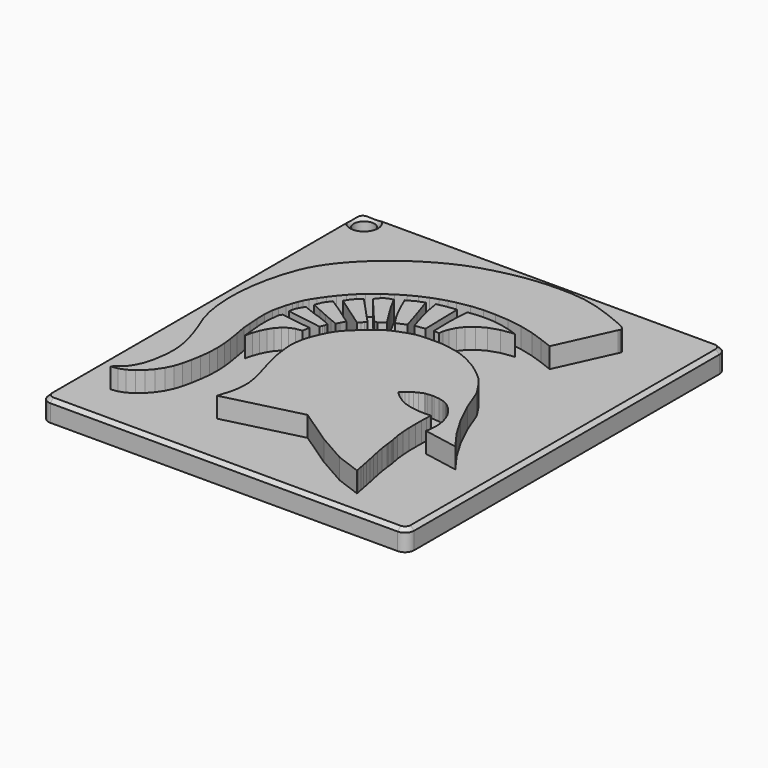
from build123d import *

# Parameters (mm, degrees)
F1_DEPTH     = 22.86
F2_W         = 203.2
F2_H         = 222.25
F2_R         = 5.715
F3_DEPTH     = 11.61275
F4_R         = 5.08
F5_T1_DEPTH  = 212.09
F5_T3_DEPTH  = 193.04
F5_T10_ANGLE = 90
F5_T12_ANGLE = 90
F5_T14_ANGLE = 90
F5_T16_ANGLE = 90


# Not quite as in the source:
# - a fillet or chamfer that OpenCascade refuses, or shapes differently, is made with other operations: its cross-section is extruded or revolved along the edge and cut away or added


with BuildPart() as f1:
    # F0 (on Top) → F1 (new body)
    with BuildSketch(Plane.XY):
        Polygon((-28.5374334, -76.846176), (-28.6309054, -77.130148), (13.3961886, -66.648838), (32.9714606, -79.89316), (49.1756446, -89.098628), (62.7590566, -94.076012), (62.6846346, -93.659706), (62.4725446, -92.483178), (62.1321846, -90.644726), (61.6787946, -88.24849), (61.1235506, -85.393022), (60.4773746, -82.180684), (59.7552526, -78.713584), (58.9681066, -75.093576), (58.1662286, -70.861428), (57.6066666, -66.742818), (57.5294506, -66.16954), (57.4758566, -65.83426), (57.4166746, -65.359026), (57.3242186, -64.361568), (57.1421006, -62.889638), (57.0415166, -62.196472), (56.8860686, -61.420756), (56.1268626, -57.560718), (55.6541686, -53.167534), (55.4100746, -48.56226), (55.3384466, -44.069762), (55.3811186, -40.012874), (55.4817026, -36.713922), (55.5850806, -34.497772), (55.6318166, -33.687512), (55.2985686, -33.722056), (54.3544506, -33.79216), (52.8840446, -33.846262), (50.9742186, -33.833816), (48.7044746, -33.701482), (46.1634586, -33.398206), (43.4334666, -32.874712), (40.5990806, -32.078168), (38.7895846, -31.333948), (37.0298726, -30.374844), (35.3803966, -29.295598), (33.8975446, -28.197556), (32.6407526, -27.172412), (31.6704726, -26.32075), (31.0451246, -25.73909), (30.8246526, -25.524206), (30.9389526, -25.358598), (31.3011566, -24.901144), (31.9435226, -24.207978), (32.8929746, -23.332948), (34.1802466, -22.331172), (35.8350566, -21.259038), (37.8868686, -20.171918), (40.3661626, -19.125946), (40.5137366, -19.106388), (40.9186126, -19.057112), (41.5165286, -18.988278), (42.2472866, -18.911062), (43.0491646, -18.833846), (43.8579006, -18.767298), (44.6145666, -18.72361), (45.2566786, -18.713704), (48.4814626, -19.051524), (51.0321306, -19.726656), (52.7105626, -20.386548), (53.3140666, -20.68576), (53.5868626, -20.857972), (54.3313366, -21.377656), (55.4281086, -22.244304), (56.7661806, -23.461218), (58.2269346, -25.02916), (59.6945466, -26.950416), (61.0544626, -29.225494), (62.1928906, -31.857696), (62.9932446, -34.675572), (63.4341886, -37.343588), (63.5942086, -39.789354), (63.5489966, -41.944798), (63.3765306, -43.740578), (63.1573286, -45.108622), (62.9686066, -45.981112), (62.8885966, -46.286928), (82.0409586, -49.814734), (74.8403126, -39.931594), (68.4324006, -29.101288), (62.7798846, -17.36344), (57.8492366, -4.759706), (57.6465446, -4.430522), (57.0872366, -3.536188), (56.2449726, -2.214626), (55.1908726, -0.606298), (53.9960566, 1.15316), (52.7367246, 2.924302), (51.4801866, 4.566666), (50.3031506, 5.943346), (49.0821726, 7.149084), (47.6171006, 8.444484), (46.0323946, 9.7536), (44.4535306, 10.997946), (43.0062386, 12.10183), (41.8172646, 12.986512), (41.0110686, 13.573506), (40.7146506, 13.78585), (40.4004526, 13.974572), (39.5378686, 14.48435), (38.2356106, 15.23111), (36.6107726, 16.131032), (34.7738446, 17.101312), (32.8393806, 18.057622), (30.9193946, 18.916396), (29.1294566, 19.594322), (27.6880066, 20.013168), (25.9600446, 20.42795), (24.0928906, 20.824952), (22.2338646, 21.185632), (20.5305406, 21.495766), (19.1302386, 21.73859), (18.1838346, 21.895562), (17.8353466, 21.95068), (17.4492666, 21.959062), (16.3702746, 21.9837), (14.7385786, 22.008338), (12.6992126, 22.018244), (10.3895906, 21.996146), (7.9519526, 21.925788), (5.5280306, 21.79066), (3.2610806, 21.574506), (1.4335506, 21.14296), (-0.5725414, 20.535646), (-2.6286714, 19.821652), (-4.6019974, 19.076162), (-6.3645034, 18.36928), (-7.7851254, 17.775174), (-8.7335614, 17.36598), (-9.0779854, 17.213072), (-9.6428814, 16.816324), (-11.1656114, 15.710916), (-13.3926834, 14.035278), (-16.0716214, 11.924284), (-18.9474094, 9.511284), (-21.7668094, 6.93293), (-24.2775994, 4.322826), (-26.2234934, 1.8161), (-27.9542494, -1.10109), (-29.5971214, -4.418076), (-31.0604154, -7.947406), (-32.2524374, -11.504168), (-32.7774554, -13.953998), (-33.1589634, -16.706088), (-33.3906114, -18.95094), (-33.4690974, -19.879818), (-33.4416654, -20.324826), (-33.3535274, -21.549868), (-33.1937614, -23.392384), (-32.9537314, -25.686766), (-32.6260714, -28.26639), (-32.2001134, -30.968696), (-31.6667134, -33.628584), (-31.0177434, -36.081462), (-30.7104034, -37.391594), (-30.2529494, -39.114222), (-29.6890694, -41.127426), (-29.0637214, -43.307762), (-28.4203394, -45.529246), (-27.8013414, -47.670466), (-27.2514314, -49.609248), (-26.8160754, -51.22037), (-26.1864094, -54.030372), (-25.7480054, -56.559196), (-25.4904494, -58.384694), (-25.4063754, -59.087512), (-25.4035814, -59.9821), (-25.4391414, -62.184026), (-25.5829054, -64.966596), (-25.8996434, -67.601084), (-26.1820914, -68.897754), (-26.5681714, -70.392798), (-27.0157194, -71.973694), (-27.4805394, -73.523856), (-27.9184354, -74.929746), (-28.2852114, -76.074778), align=None)
    extrude(amount=F1_DEPTH)


with BuildPart() as f1b:
    # F0 (on Top) → F1, piece 2 (new body)
    with BuildSketch(Plane.XY):
        Polygon((-55.0672254, -19.514566), (-54.5256974, -25.240234), (-53.4987754, -21.424646), (-52.2559534, -17.902174), (-50.7537974, -14.729968), (-48.9501434, -11.96975), (-46.8018114, -9.678162), (-44.2648594, -7.915656), (-41.2950914, -6.740144), (-37.8485654, -6.211062), (-37.1348254, -2.21869), (-53.8833314, 0.132334), (-54.8109394, -0.865378), (-55.6473614, -7.671562), (-55.5866554, -13.773404), align=None)
    extrude(amount=F1_DEPTH)


with BuildPart() as f1c:
    # F0 (on Top) → F1, piece 3 (new body)
    with BuildSketch(Plane.XY):
        Polygon((-53.6326334, 5.551932), (-53.8132274, 4.480052), (-34.4269314, 1.34493), (-33.8414614, 2.590546), (-33.4746854, 3.615944), (-33.2473554, 4.503166), (-33.0723494, 5.335778), (-35.2277934, 6.342888), (-37.6199654, 7.368032), (-40.4640034, 8.429244), (-43.9765694, 9.54024), (-50.6765814, 12.177522), (-52.3867634, 9.326372), (-53.0662134, 7.85876), (-53.4327354, 6.639306), align=None)
    extrude(amount=F1_DEPTH)


with BuildPart() as f1d:
    # F0 (on Top) → F1, piece 4 (new body)
    with BuildSketch(Plane.XY):
        Polygon((-40.1444714, 20.660868), (-44.7609214, 23.652734), (-47.4703394, 20.017232), (-49.0382814, 15.954756), (-44.0540394, 13.701776), (-39.1424414, 11.495532), (-34.5991434, 9.523476), (-30.7213254, 7.97306), (-30.4965354, 8.382254), (-30.2940974, 8.743696), (-30.0916594, 9.10209), (-29.8696634, 9.504172), (-29.6080434, 9.9949), (-29.2841934, 10.621772), (-28.8788094, 11.429238), (-28.3690314, 12.463018), (-32.2013834, 15.161006), (-36.0418634, 17.862296), align=None)
    extrude(amount=F1_DEPTH)


with BuildPart() as f1e:
    # F0 (on Top) → F1, piece 5 (new body)
    with BuildSketch(Plane.XY):
        Polygon((-40.5564594, 28.533852), (-41.6959034, 26.717244), (-24.0929414, 14.529816), (-22.8099874, 15.813024), (-21.7061034, 16.84655), (-21.0284314, 18.022062), (-35.5678994, 33.631124), (-37.6489214, 32.02559), (-39.2582654, 30.313884), align=None)
    extrude(amount=F1_DEPTH)


with BuildPart() as f1f:
    # F0 (on Top) → F1, piece 6 (new body)
    with BuildSketch(Plane.XY):
        Polygon((-22.1058994, 35.819334), (-25.0190254, 41.327324), (-27.6359874, 40.711374), (-29.6342054, 39.529004), (-31.2135774, 37.963602), (-32.5734934, 36.196778), (-19.2466214, 20.302728), (-18.5366914, 20.20316), (-18.0157374, 20.166076), (-17.5956214, 20.162012), (-17.1793154, 20.160488), (-13.9009374, 22.511512), (-16.6253414, 26.879804), (-19.3332354, 31.160212), align=None)
    extrude(amount=F1_DEPTH)


with BuildPart() as f1g:
    # F0 (on Top) → F1, piece 7 (new body)
    with BuildSketch(Plane.XY):
        Polygon((-9.0904314, 37.43706), (-12.4747274, 47.813722), (-16.6819834, 46.238668), (-21.0284314, 43.822874), (-18.7132214, 38.437566), (-16.2877754, 33.349946), (-13.7205974, 28.653232), (-10.9781594, 24.436578), (-5.7046114, 26.573988), align=None)
    extrude(amount=F1_DEPTH)


with BuildPart() as f1h:
    # F0 (on Top) → F1, piece 8 (new body)
    with BuildSketch(Plane.XY):
        Polygon((-5.3119274, 50.035206), (-8.1986374, 49.452022), (-7.1417434, 43.384724), (-5.8425334, 37.846254), (-4.3678094, 32.695134), (-2.7818334, 27.786584), (2.7774646, 28.570682), (2.2786086, 51.0921), (2.1752306, 51.094894), (1.8333466, 51.086512), (1.2008866, 51.04384), (0.2224786, 50.940462), (-1.1544554, 50.754534), (-2.9814774, 50.46091), align=None)
    extrude(amount=F1_DEPTH)


with BuildPart() as f1i:
    # F0 (on Top) → F1, piece 9 (new body)
    with BuildSketch(Plane.XY):
        Polygon((6.7680586, 34.653474), (6.9115686, 29.139896), (9.9044506, 28.99791), (10.2709726, 31.41091), (11.1805466, 34.291016), (12.7736346, 37.417756), (15.1962866, 40.570912), (18.5917586, 43.52798), (23.1048306, 46.070266), (28.8787586, 47.976282), (36.0611166, 49.024794), (33.2716886, 49.884838), (30.4494946, 50.724054), (27.4964906, 51.484784), (24.3148866, 52.105052), (20.8061306, 52.529232), (16.8719246, 52.69484), (12.4152406, 52.544472), (7.3387966, 52.018184), (6.8589906, 45.99051), (6.7101466, 40.235632), align=None)
    extrude(amount=F1_DEPTH)


with BuildPart() as f1j:
    # F0 (on Top) → F1, piece 10 (new body)
    with BuildSketch(Plane.XY):
        Polygon((-80.1116762, -82.471768), (-81.8232298, -84.466938), (-78.2404074, -84.005166), (-74.6808514, -82.658966), (-71.2439774, -80.545178), (-68.0275754, -77.780896), (-65.1324834, -74.48169), (-62.6562374, -70.765162), (-60.6994214, -66.747898), (-59.3598254, -62.547754), (-58.2836274, -57.613296), (-57.3821814, -52.464716), (-56.7761374, -47.191168), (-56.5830974, -41.882822), (-56.8449714, -36.6903), (-57.4690494, -31.55315), (-58.3717654, -26.07945), (-59.4741254, -19.879818), (-59.7979754, -15.06601), (-60.1934534, -9.724898), (-60.3341694, -4.328668), (-59.8970354, 0.65024), (-59.2165694, 3.894328), (-58.1746614, 7.818882), (-57.1660274, 11.035284), (-56.4025034, 13.211302), (-56.1010054, 14.009116), (-55.3247814, 15.939516), (-53.8932374, 18.549874), (-51.9211814, 21.650452), (-49.5234214, 25.049988), (-46.8155274, 28.562554), (-43.9092594, 31.99511), (-40.9229814, 35.160712), (-37.9699774, 37.867082), (-32.8531474, 41.883838), (-27.9156414, 45.29074), (-23.1559354, 48.14443), (-18.5752994, 50.506376), (-14.1767814, 52.430172), (-9.9611434, 53.977794), (-5.9278774, 55.202582), (-2.0774914, 56.166004), (4.8267366, 57.417462), (11.4340386, 57.97931), (18.1630066, 57.961784), (25.4324866, 57.469532), (33.7212686, 56.274716), (41.2190946, 54.399434), (48.2386386, 52.038504), (55.0902886, 49.381918), (68.9175406, 79.743046), (69.0734966, 79.970122), (69.3709306, 80.536796), (69.5487306, 81.276444), (69.3447686, 82.023712), (69.0127906, 82.38871), (68.5357786, 82.773266), (67.9724066, 83.157568), (67.3810946, 83.518756), (66.8187386, 83.835494), (66.3460446, 84.08924), (66.0194006, 84.257388), (65.8984966, 84.316824), (56.3402226, 88.194388), (47.7192086, 91.15044), (39.5406626, 93.101668), (31.3125866, 93.968316), (24.6704866, 94.076012), (18.5310526, 93.918532), (12.7916686, 93.512132), (7.3525126, 92.865956), (2.1102066, 91.99626), (-3.0340554, 90.913204), (-8.1811114, 89.62898), (-13.4325614, 88.158574), (-17.9606194, 86.675722), (-22.5730054, 84.855304), (-27.2349214, 82.719418), (-31.9052194, 80.295496), (-36.5465614, 77.606906), (-41.1216094, 74.675746), (-45.5917554, 71.529702), (-49.9173754, 68.189602), (-54.0611314, 64.680846), (-57.9859394, 61.027818), (-61.6514134, 57.256172), (-65.0194534, 53.386482), (-68.0522134, 49.446688), (-70.7133714, 45.458634), (-72.9610174, 41.447212), (-74.7593374, 37.43579), (-77.5500354, 29.324554), (-79.6679636, 21.099018), (-81.1190402, 12.8778), (-81.90865, 4.773422), (-82.0409586, -3.098038), (-81.521427, -10.622026), (-80.3542208, -17.684496), (-78.5449534, -24.170894), (-75.5739154, -31.693612), (-73.3509074, -38.023038), (-71.7827114, -43.34891), (-70.7700134, -47.861982), (-70.2201034, -51.753516), (-70.0326514, -55.214012), (-70.1126614, -58.431684), (-70.3620894, -61.599826), (-71.2757274, -67.696334), (-72.6110054, -72.501506), (-74.2025694, -76.162916), (-75.8825254, -78.827884), (-77.4809474, -80.642968), (-78.8301954, -81.75625), (-79.7644074, -82.317082), align=None)
    extrude(amount=F1_DEPTH)


with BuildPart() as f3:
    # F2 (on face) → F3 (new body)
    with BuildSketch(Plane(origin=(0, 0, 0), x_dir=(1, 0, 0), z_dir=(0, 0, -1))):
        with Locations((0, -3.175)):
            Rectangle(F2_W, F2_H)
        with Locations((-93.472, -106.172)):
            Circle(F2_R, mode=Mode.SUBTRACT)
        Polygon((-5.7046114, -26.573988), (-9.0904314, -37.43706), (-12.4747274, -47.813722), (-16.6819834, -46.238668), (-21.0284314, -43.822874), (-18.7132214, -38.437566), (-16.2877754, -33.349946), (-13.7205974, -28.653232), (-10.9781594, -24.436578), align=None, mode=Mode.SUBTRACT)
        Polygon((-2.9814774, -50.46091), (-5.3119274, -50.035206), (-8.1986374, -49.452022), (-7.1417434, -43.384724), (-5.8425334, -37.846254), (-4.3678094, -32.695134), (-2.7818334, -27.786584), (2.7774646, -28.570682), (2.2786086, -51.0921), (2.1752306, -51.094894), (1.8333466, -51.086512), (1.2008866, -51.04384), (0.2224786, -50.940462), (-1.1544554, -50.754534), align=None, mode=Mode.SUBTRACT)
        Polygon((-39.2582654, -30.313884), (-40.5564594, -28.533852), (-41.6959034, -26.717244), (-24.0929414, -14.529816), (-22.8099874, -15.813024), (-21.7061034, -16.84655), (-21.0284314, -18.022062), (-35.5678994, -33.631124), (-37.6489214, -32.02559), align=None, mode=Mode.SUBTRACT)
        Polygon((-36.0418634, -17.862296), (-40.1444714, -20.660868), (-44.7609214, -23.652734), (-47.4703394, -20.017232), (-49.0382814, -15.954756), (-44.0540394, -13.701776), (-39.1424414, -11.495532), (-34.5991434, -9.523476), (-30.7213254, -7.97306), (-30.4965354, -8.382254), (-30.2940974, -8.743696), (-30.0916594, -9.10209), (-29.8696634, -9.504172), (-29.6080434, -9.9949), (-29.2841934, -10.621772), (-28.8788094, -11.429238), (-28.3690314, -12.463018), (-32.2013834, -15.161006), align=None, mode=Mode.SUBTRACT)
        Polygon((-53.8132274, -4.480052), (-34.4269314, -1.34493), (-33.8414614, -2.590546), (-33.4746854, -3.615944), (-33.2473554, -4.503166), (-33.0723494, -5.335778), (-35.2277934, -6.342888), (-37.6199654, -7.368032), (-40.4640034, -8.429244), (-43.9765694, -9.54024), (-50.6765814, -12.177522), (-52.3867634, -9.326372), (-53.0662134, -7.85876), (-53.4327354, -6.639306), (-53.6326334, -5.551932), align=None, mode=Mode.SUBTRACT)
        Polygon((-19.3332354, -31.160212), (-22.1058994, -35.819334), (-25.0190254, -41.327324), (-27.6359874, -40.711374), (-29.6342054, -39.529004), (-31.2135774, -37.963602), (-32.5734934, -36.196778), (-19.2466214, -20.302728), (-18.5366914, -20.20316), (-18.0157374, -20.166076), (-17.5956214, -20.162012), (-17.1793154, -20.160488), (-13.9009374, -22.511512), (-16.6253414, -26.879804), align=None, mode=Mode.SUBTRACT)
        Polygon((-79.7644074, 82.317082), (-80.1116762, 82.471768), (-81.8232298, 84.466938), (-78.2404074, 84.005166), (-74.6808514, 82.658966), (-71.2439774, 80.545178), (-68.0275754, 77.780896), (-65.1324834, 74.48169), (-62.6562374, 70.765162), (-60.6994214, 66.747898), (-59.3598254, 62.547754), (-58.2836274, 57.613296), (-57.3821814, 52.464716), (-56.7761374, 47.191168), (-56.5830974, 41.882822), (-56.8449714, 36.6903), (-57.4690494, 31.55315), (-58.3717654, 26.07945), (-59.4741254, 19.879818), (-59.7979754, 15.06601), (-60.1934534, 9.724898), (-60.3341694, 4.328668), (-59.8970354, -0.65024), (-59.2165694, -3.894328), (-58.1746614, -7.818882), (-57.1660274, -11.035284), (-56.4025034, -13.211302), (-56.1010054, -14.009116), (-55.3247814, -15.939516), (-53.8932374, -18.549874), (-51.9211814, -21.650452), (-49.5234214, -25.049988), (-46.8155274, -28.562554), (-43.9092594, -31.99511), (-40.9229814, -35.160712), (-37.9699774, -37.867082), (-32.8531474, -41.883838), (-27.9156414, -45.29074), (-23.1559354, -48.14443), (-18.5752994, -50.506376), (-14.1767814, -52.430172), (-9.9611434, -53.977794), (-5.9278774, -55.202582), (-2.0774914, -56.166004), (4.8267366, -57.417462), (11.4340386, -57.97931), (18.1630066, -57.961784), (25.4324866, -57.469532), (33.7212686, -56.274716), (41.2190946, -54.399434), (48.2386386, -52.038504), (55.0902886, -49.381918), (68.9175406, -79.743046), (69.0734966, -79.970122), (69.3709306, -80.536796), (69.5487306, -81.276444), (69.3447686, -82.023712), (69.0127906, -82.38871), (68.5357786, -82.773266), (67.9724066, -83.157568), (67.3810946, -83.518756), (66.8187386, -83.835494), (66.3460446, -84.08924), (66.0194006, -84.257388), (65.8984966, -84.316824), (56.3402226, -88.194388), (47.7192086, -91.15044), (39.5406626, -93.101668), (31.3125866, -93.968316), (24.6704866, -94.076012), (18.5310526, -93.918532), (12.7916686, -93.512132), (7.3525126, -92.865956), (2.1102066, -91.99626), (-3.0340554, -90.913204), (-8.1811114, -89.62898), (-13.4325614, -88.158574), (-17.9606194, -86.675722), (-22.5730054, -84.855304), (-27.2349214, -82.719418), (-31.9052194, -80.295496), (-36.5465614, -77.606906), (-41.1216094, -74.675746), (-45.5917554, -71.529702), (-49.9173754, -68.189602), (-54.0611314, -64.680846), (-57.9859394, -61.027818), (-61.6514134, -57.256172), (-65.0194534, -53.386482), (-68.0522134, -49.446688), (-70.7133714, -45.458634), (-72.9610174, -41.447212), (-74.7593374, -37.43579), (-77.5500354, -29.324554), (-79.6679636, -21.099018), (-81.1190402, -12.8778), (-81.90865, -4.773422), (-82.0409586, 3.098038), (-81.521427, 10.622026), (-80.3542208, 17.684496), (-78.5449534, 24.170894), (-75.5739154, 31.693612), (-73.3509074, 38.023038), (-71.7827114, 43.34891), (-70.7700134, 47.861982), (-70.2201034, 51.753516), (-70.0326514, 55.214012), (-70.1126614, 58.431684), (-70.3620894, 61.599826), (-71.2757274, 67.696334), (-72.6110054, 72.501506), (-74.2025694, 76.162916), (-75.8825254, 78.827884), (-77.4809474, 80.642968), (-78.8301954, 81.75625), align=None, mode=Mode.SUBTRACT)
        Polygon((6.7101466, -40.235632), (6.7680586, -34.653474), (6.9115686, -29.139896), (9.9044506, -28.99791), (10.2709726, -31.41091), (11.1805466, -34.291016), (12.7736346, -37.417756), (15.1962866, -40.570912), (18.5917586, -43.52798), (23.1048306, -46.070266), (28.8787586, -47.976282), (36.0611166, -49.024794), (33.2716886, -49.884838), (30.4494946, -50.724054), (27.4964906, -51.484784), (24.3148866, -52.105052), (20.8061306, -52.529232), (16.8719246, -52.69484), (12.4152406, -52.544472), (7.3387966, -52.018184), (6.8589906, -45.99051), align=None, mode=Mode.SUBTRACT)
        Polygon((-55.5866554, 13.773404), (-55.0672254, 19.514566), (-54.5256974, 25.240234), (-53.4987754, 21.424646), (-52.2559534, 17.902174), (-50.7537974, 14.729968), (-48.9501434, 11.96975), (-46.8018114, 9.678162), (-44.2648594, 7.915656), (-41.2950914, 6.740144), (-37.8485654, 6.211062), (-37.1348254, 2.21869), (-53.8833314, -0.132334), (-54.8109394, 0.865378), (-55.6473614, 7.671562), align=None, mode=Mode.SUBTRACT)
        Polygon((-28.2852114, 76.074778), (-28.5374334, 76.846176), (-28.6309054, 77.130148), (13.3961886, 66.648838), (32.9714606, 79.89316), (49.1756446, 89.098628), (62.7590566, 94.076012), (62.6846346, 93.659706), (62.4725446, 92.483178), (62.1321846, 90.644726), (61.6787946, 88.24849), (61.1235506, 85.393022), (60.4773746, 82.180684), (59.7552526, 78.713584), (58.9681066, 75.093576), (58.1662286, 70.861428), (57.6066666, 66.742818), (57.5294506, 66.16954), (57.4758566, 65.83426), (57.4166746, 65.359026), (57.3242186, 64.361568), (57.1421006, 62.889638), (57.0415166, 62.196472), (56.8860686, 61.420756), (56.1268626, 57.560718), (55.6541686, 53.167534), (55.4100746, 48.56226), (55.3384466, 44.069762), (55.3811186, 40.012874), (55.4817026, 36.713922), (55.5850806, 34.497772), (55.6318166, 33.687512), (55.2985686, 33.722056), (54.3544506, 33.79216), (52.8840446, 33.846262), (50.9742186, 33.833816), (48.7044746, 33.701482), (46.1634586, 33.398206), (43.4334666, 32.874712), (40.5990806, 32.078168), (38.7895846, 31.333948), (37.0298726, 30.374844), (35.3803966, 29.295598), (33.8975446, 28.197556), (32.6407526, 27.172412), (31.6704726, 26.32075), (31.0451246, 25.73909), (30.8246526, 25.524206), (30.9389526, 25.358598), (31.3011566, 24.901144), (31.9435226, 24.207978), (32.8929746, 23.332948), (34.1802466, 22.331172), (35.8350566, 21.259038), (37.8868686, 20.171918), (40.3661626, 19.125946), (40.5137366, 19.106388), (40.9186126, 19.057112), (41.5165286, 18.988278), (42.2472866, 18.911062), (43.0491646, 18.833846), (43.8579006, 18.767298), (44.6145666, 18.72361), (45.2566786, 18.713704), (48.4814626, 19.051524), (51.0321306, 19.726656), (52.7105626, 20.386548), (53.3140666, 20.68576), (53.5868626, 20.857972), (54.3313366, 21.377656), (55.4281086, 22.244304), (56.7661806, 23.461218), (58.2269346, 25.02916), (59.6945466, 26.950416), (61.0544626, 29.225494), (62.1928906, 31.857696), (62.9932446, 34.675572), (63.4341886, 37.343588), (63.5942086, 39.789354), (63.5489966, 41.944798), (63.3765306, 43.740578), (63.1573286, 45.108622), (62.9686066, 45.981112), (62.8885966, 46.286928), (82.0409586, 49.814734), (74.8403126, 39.931594), (68.4324006, 29.101288), (62.7798846, 17.36344), (57.8492366, 4.759706), (57.6465446, 4.430522), (57.0872366, 3.536188), (56.2449726, 2.214626), (55.1908726, 0.606298), (53.9960566, -1.15316), (52.7367246, -2.924302), (51.4801866, -4.566666), (50.3031506, -5.943346), (49.0821726, -7.149084), (47.6171006, -8.444484), (46.0323946, -9.7536), (44.4535306, -10.997946), (43.0062386, -12.10183), (41.8172646, -12.986512), (41.0110686, -13.573506), (40.7146506, -13.78585), (40.4004526, -13.974572), (39.5378686, -14.48435), (38.2356106, -15.23111), (36.6107726, -16.131032), (34.7738446, -17.101312), (32.8393806, -18.057622), (30.9193946, -18.916396), (29.1294566, -19.594322), (27.6880066, -20.013168), (25.9600446, -20.42795), (24.0928906, -20.824952), (22.2338646, -21.185632), (20.5305406, -21.495766), (19.1302386, -21.73859), (18.1838346, -21.895562), (17.8353466, -21.95068), (17.4492666, -21.959062), (16.3702746, -21.9837), (14.7385786, -22.008338), (12.6992126, -22.018244), (10.3895906, -21.996146), (7.9519526, -21.925788), (5.5280306, -21.79066), (3.2610806, -21.574506), (1.4335506, -21.14296), (-0.5725414, -20.535646), (-2.6286714, -19.821652), (-4.6019974, -19.076162), (-6.3645034, -18.36928), (-7.7851254, -17.775174), (-8.7335614, -17.36598), (-9.0779854, -17.213072), (-9.6428814, -16.816324), (-11.1656114, -15.710916), (-13.3926834, -14.035278), (-16.0716214, -11.924284), (-18.9474094, -9.511284), (-21.7668094, -6.93293), (-24.2775994, -4.322826), (-26.2234934, -1.8161), (-27.9542494, 1.10109), (-29.5971214, 4.418076), (-31.0604154, 7.947406), (-32.2524374, 11.504168), (-32.7774554, 13.953998), (-33.1589634, 16.706088), (-33.3906114, 18.95094), (-33.4690974, 19.879818), (-33.4416654, 20.324826), (-33.3535274, 21.549868), (-33.1937614, 23.392384), (-32.9537314, 25.686766), (-32.6260714, 28.26639), (-32.2001134, 30.968696), (-31.6667134, 33.628584), (-31.0177434, 36.081462), (-30.7104034, 37.391594), (-30.2529494, 39.114222), (-29.6890694, 41.127426), (-29.0637214, 43.307762), (-28.4203394, 45.529246), (-27.8013414, 47.670466), (-27.2514314, 49.609248), (-26.8160754, 51.22037), (-26.1864094, 54.030372), (-25.7480054, 56.559196), (-25.4904494, 58.384694), (-25.4063754, 59.087512), (-25.4035814, 59.9821), (-25.4391414, 62.184026), (-25.5829054, 64.966596), (-25.8996434, 67.601084), (-26.1820914, 68.897754), (-26.5681714, 70.392798), (-27.0157194, 71.973694), (-27.4805394, 73.523856), (-27.9184354, 74.929746), align=None, mode=Mode.SUBTRACT)
    extrude(amount=-F3_DEPTH)

    # F4
    f4_edges = [f3.edges().sort_by_distance(p)[0] for p in [
        (-101.6, 114.3, 5.806375),
        (-101.6, -107.95, 5.806375),
        (101.6, -107.95, 5.806375),
        (101.6, 114.3, 5.806375),
    ]]
    fillet(f4_edges, radius=F4_R)

    # F5: chamfer of 2.032 on 3 edges, made by hand

    # F5_s2 → F5_t1 (cut)
    with BuildSketch(Plane.XZ.offset(-109.22)):
        Polygon((99.568, 11.61275), (101.6, 9.58075), (101.6, 11.61275), align=None)
        Polygon((-101.6, 9.58075), (-99.568, 11.61275), (-101.6, 11.61275), align=None)
    extrude(amount=F5_T1_DEPTH, mode=Mode.SUBTRACT)

    # F5_s4 → F5_t3 (cut)
    with BuildSketch(Plane.YZ.offset(-96.52)):
        Polygon((-105.918, 11.61275), (-107.95, 9.58075), (-107.95, 11.61275), align=None)
        Polygon((112.268, 11.61275), (114.3, 9.58075), (114.3, 11.61275), align=None)
    extrude(amount=F5_T3_DEPTH, mode=Mode.SUBTRACT)

    # F5_s5 → F5_t6 (revolve, cut)
    with BuildSketch(Plane.XZ.offset(-106.172)):
        Polygon((-85.725, 11.61275), (-87.757, 9.58075), (-87.757, 11.61275), align=None)
    revolve(axis=Axis((-93.472, 106.172, 11.61275), (0, 0, -1)), mode=Mode.SUBTRACT)

    # F5_s7 → F5_t8 (revolve, cut)
    with BuildSketch(Plane.XZ.offset(-106.172)):
        Polygon((-85.725, 0), (-87.757, 2.032), (-87.757, 0), align=None)
    revolve(axis=Axis((-93.472, 106.172, 0), (0, 0, -1)), mode=Mode.SUBTRACT)

    # F5_s9 → F5_t10 (revolve, cut)
    with BuildSketch(Plane.YZ.offset(96.52)):
        Polygon((112.268, 11.61275), (114.3, 9.58075), (114.3, 11.61275), align=None)
    revolve(axis=Axis((96.52, 109.22, 11.61275), (0, 0, -1)), revolution_arc=F5_T10_ANGLE, mode=Mode.SUBTRACT)

    # F5_s11 → F5_t12 (revolve, cut)
    with BuildSketch(Plane.XZ.offset(102.87)):
        Polygon((99.568, 11.61275), (101.6, 9.58075), (101.6, 11.61275), align=None)
    revolve(axis=Axis((96.52, -102.87, 11.61275), (0, 0, -1)), revolution_arc=F5_T12_ANGLE, mode=Mode.SUBTRACT)

    # F5_s13 → F5_t14 (revolve, cut)
    with BuildSketch(Plane.XZ.offset(102.87)):
        Polygon((-101.6, 9.58075), (-99.568, 11.61275), (-101.6, 11.61275), align=None)
    revolve(axis=Axis((-96.52, -102.87, 11.61275), (0, 0, 1)), revolution_arc=F5_T14_ANGLE, mode=Mode.SUBTRACT)

    # F5_s15 → F5_t16 (revolve, cut)
    with BuildSketch(Plane.XZ.offset(-109.22)):
        Polygon((-101.6, 9.58075), (-99.568, 11.61275), (-101.6, 11.61275), align=None)
    revolve(axis=Axis((-96.52, 109.22, 11.61275), (0, 0, -1)), revolution_arc=F5_T16_ANGLE, mode=Mode.SUBTRACT)


solid = Compound([f1.part, f1b.part, f1c.part, f1d.part, f1e.part, f1f.part, f1g.part, f1h.part, f1i.part, f1j.part, f3.part])
